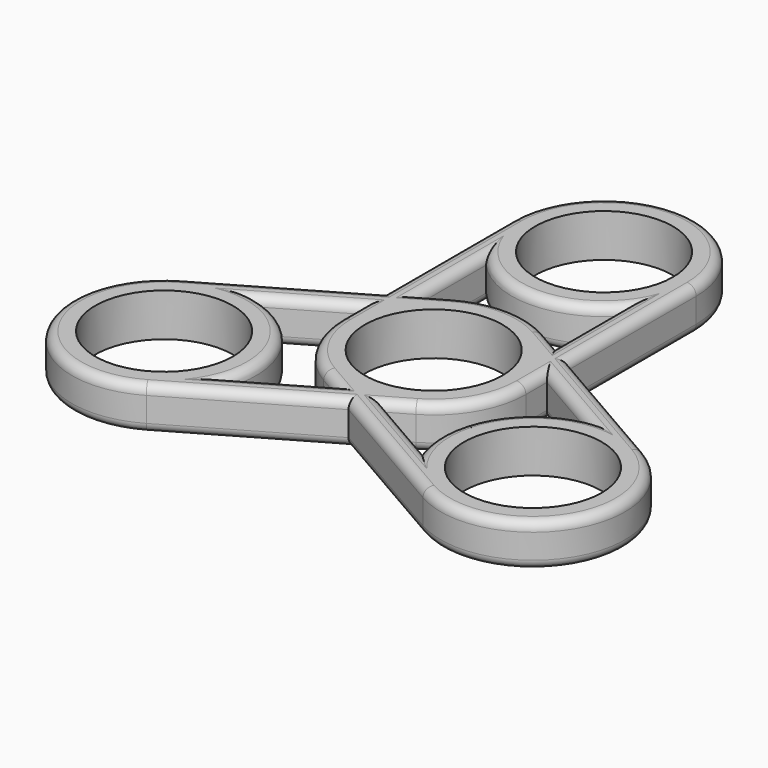
from build123d import *

# Parameters (mm, degrees)
F0_R     = 11.2
F1_DEPTH = 7
F2_R     = 1.5
F3_R     = 1.49999
F4_R     = 1.49999


# Not quite as in the source:
# - a fillet or chamfer is up to 0.001 mm smaller than in the source, because OpenCascade refuses the exact size


with BuildPart() as f1:
    # F0 (on Top) → F1 (new body)
    with BuildSketch(Plane.XY):
        with BuildLine():
            Line((-15, 8.6602540378), (-37.5131404032, -4.3377136343))
            ThreePointArc((-37.5131404032, -4.3377136343), (-43.00352146, -24.828094691), (-22.5131404032, -30.3184757478))
            Line((-22.5131404032, -30.3184757478), (0, -17.3205080757))
            Line((0, -17.3205080757), (22.5131404032, -30.3184757478))
            ThreePointArc((22.5131404032, -30.3184757478), (43.00352146, -24.828094691), (37.5131404032, -4.3377136343))
            Line((37.5131404032, -4.3377136343), (15, 8.6602540378))
            Line((15, 8.6602540378), (15, 34.6561893821))
            ThreePointArc((15, 34.6561893821), (0, 49.6561893821), (-15, 34.6561893821))
            Line((-15, 34.6561893821), (-15, 8.6602540378))
        make_face()
        with Locations((-30.0131404032, -17.328094691)):
            Circle(F0_R, mode=Mode.SUBTRACT)
        with BuildLine():
            Line((-15, 4.272391992), (-15, 0))
            ThreePointArc((-15, 0), (-12.9903810568, -7.5), (-7.5, -12.9903810568))
            Line((-7.5, -12.9903810568), (-3.8, -15.1265770528))
            Line((-3.8, -15.1265770528), (-15.7719599283, -22.0385913401))
            ThreePointArc((-15.7719599283, -22.0385913401), (-17.0227593465, -9.828094691), (-26.9719599283, -2.6396222953))
            Line((-26.9719599283, -2.6396222953), (-15, 4.272391992))
        make_face(mode=Mode.SUBTRACT)
        with Locations((30.0131404032, -17.328094691)):
            Circle(F0_R, mode=Mode.SUBTRACT)
        with BuildLine():
            ThreePointArc((26.9719599283, -2.6396222953), (17.0227593465, -9.828094691), (15.7719599283, -22.0385913401))
            Line((15.7719599283, -22.0385913401), (3.8, -15.1265770528))
            Line((3.8, -15.1265770528), (7.5, -12.9903810568))
            ThreePointArc((7.5, -12.9903810568), (12.9903810568, -7.5), (15, 0))
            Line((15, 0), (15, 4.272391992))
            Line((15, 4.272391992), (26.9719599283, -2.6396222953))
        make_face(mode=Mode.SUBTRACT)
        Circle(F0_R, mode=Mode.SUBTRACT)
        with BuildLine():
            Line((-11.2, 10.8541850608), (-11.2, 24.6782136355))
            ThreePointArc((-11.2, 24.6782136355), (0, 19.6561893821), (11.2, 24.6782136355))
            Line((11.2, 24.6782136355), (11.2, 10.8541850608))
            Line((11.2, 10.8541850608), (7.5, 12.9903810568))
            ThreePointArc((7.5, 12.9903810568), (0, 15), (-7.5, 12.9903810568))
            Line((-7.5, 12.9903810568), (-11.2, 10.8541850608))
        make_face(mode=Mode.SUBTRACT)
        with BuildLine():
            ThreePointArc((-11.2, 34.6561893821), (0, 45.8561893821), (11.2, 34.6561893821))
            ThreePointArc((11.2, 34.6561893821), (0, 23.4561893821), (-11.2, 34.6561893821))
        make_face(mode=Mode.SUBTRACT)
    extrude(amount=F1_DEPTH)

    # F2
    f2_edges = [f1.edges().sort_by_distance(p)[0] for p in [
        (-15, 21.658222, 7),
        (-26.25657, 2.16127, 7),
        (11.25657, -23.819492, 7),
        (15, 21.658222, 0),
        (26.25657, 2.16127, 0),
        (-11.25657, -23.819492, 0),
    ]]
    fillet(f2_edges, radius=F2_R)

    # F3 (radius 1.5 in the source; OpenCascade refuses exactly that, so slightly less here)
    f3_edges = [f1.edges().sort_by_distance(p)[0] for p in [
        (17.022759, -9.828095, 7),
        (9.78598, -18.582584, 7),
        (20.98598, 0.816385, 7),
        (12.990381, -7.5, 7),
        (5.65, -14.058479, 7),
        (15, 2.136196, 7),
        (-20.98598, 0.816385, 7),
        (-17.022759, -9.828095, 7),
        (-9.78598, -18.582584, 7),
        (-12.990381, -7.5, 7),
        (-5.65, -14.058479, 7),
        (-15, 2.136196, 7),
        (0, 19.656189, 7),
        (-11.2, 17.766199, 7),
        (11.2, 17.766199, 7),
        (0, 15, 7),
        (9.35, 11.922283, 7),
        (-9.35, 11.922283, 7),
    ]]
    fillet(f3_edges, radius=F3_R)

    # F4 (radius 1.5 in the source; OpenCascade refuses exactly that, so slightly less here)
    f4_edges = [f1.edges().sort_by_distance(p)[0] for p in [
        (-17.022759, -9.828095, 0),
        (-9.78598, -18.582584, 0),
        (-20.98598, 0.816385, 0),
        (-11.2, 17.766199, 0),
        (0, 19.656189, 0),
        (11.2, 17.766199, 0),
        (17.022759, -9.828095, 0),
        (20.98598, 0.816385, 0),
        (9.78598, -18.582584, 0),
        (-12.990381, -7.5, 0),
        (-5.65, -14.058479, 0),
        (-15, 2.136196, 0),
        (-9.35, 11.922283, 0),
        (0, 15, 0),
        (9.35, 11.922283, 0),
        (15, 2.136196, 0),
        (12.990381, -7.5, 0),
        (5.65, -14.058479, 0),
    ]]
    fillet(f4_edges, radius=F4_R)


solid = f1.part
